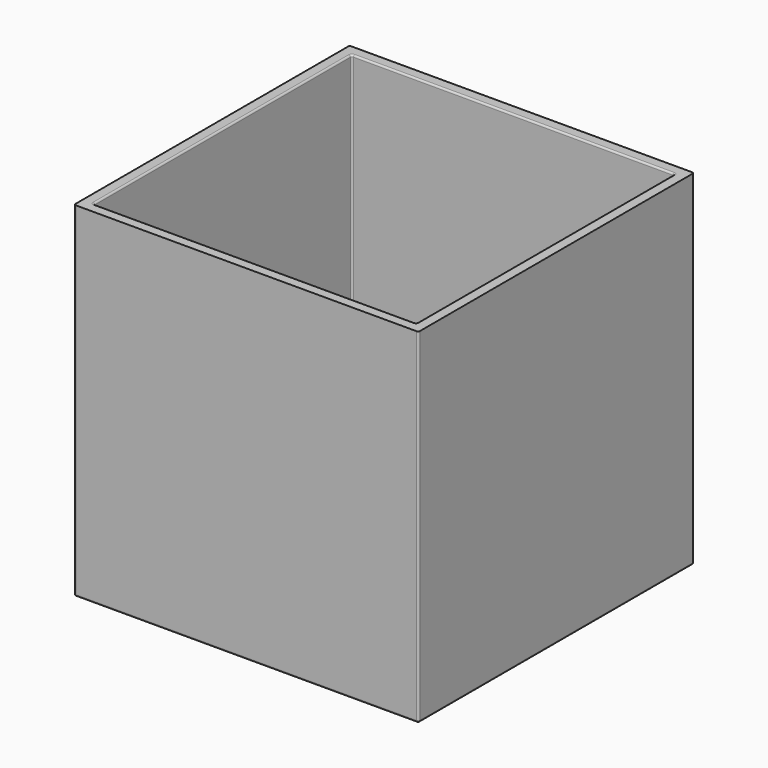
from build123d import *

# Parameters (mm, degrees)
F0_W         = 50.8
F0_H         = 50.8
F1_DEPTH     = 1.5875
F2_W         = 50.8
F2_H         = 50.8
F2_W_2       = 47.625
F2_H_2       = 47.625
F3_DEPTH     = 49.2125
F4_R         = 0.254
F5_TEXT_SIZE = 5.9603176266
F6_DEPTH     = 0.254


# Not quite as in the source:
# - Text() gives the source's letters only with a copy of the font that has no kerning and outlines rounded to 1/6400 em; it was checked with that copy


with BuildPart() as f1:
    # F0 (on Top) → F1 (new body)
    with BuildSketch(Plane.XY):
        Rectangle(F0_W, F0_H)
    extrude(amount=F1_DEPTH)

    # F2 (on face) → F3 (join)
    with BuildSketch(Plane.XY.offset(1.5875)):
        Rectangle(F2_W, F2_H)
        Rectangle(F2_W_2, F2_H_2, mode=Mode.SUBTRACT)
    extrude(amount=F3_DEPTH)

    # F4
    f4_edges = [f1.edges().sort_by_distance(p)[0] for p in [
        (-23.8125, 0, 1.5875),
        (-23.8125, -23.8125, 26.19375),
        (0, -23.8125, 1.5875),
        (-23.8125, 0, 50.8),
        (0, -23.8125, 50.8),
        (0, 23.8125, 1.5875),
        (-23.8125, 23.8125, 26.19375),
        (0, 23.8125, 50.8),
        (23.8125, 23.8125, 26.19375),
        (23.8125, 0, 1.5875),
        (23.8125, 0, 50.8),
        (23.8125, -23.8125, 26.19375),
        (-25.4, -25.4, 25.4),
        (25.4, -25.4, 25.4),
        (25.4, 25.4, 25.4),
        (-25.4, 25.4, 25.4),
        (-25.4, 0, 0),
        (0, -25.4, 0),
        (0, 25.4, 0),
        (25.4, 0, 0),
    ]]
    fillet(f4_edges, radius=F4_R)

    # F5 (on face) → F6 (cut)
    with BuildSketch(Plane(origin=(0, 25.4, 0), x_dir=(-1, 0, 0), z_dir=(0, 1, 0))):
        with Locations((-22.225, 33.8085713088)):
            Text('APP Connectors', F5_TEXT_SIZE, font='Open Sans', text_align=(TextAlign.LEFT, TextAlign.BOTTOM))
    extrude(amount=-F6_DEPTH, mode=Mode.SUBTRACT)


solid = f1.part
